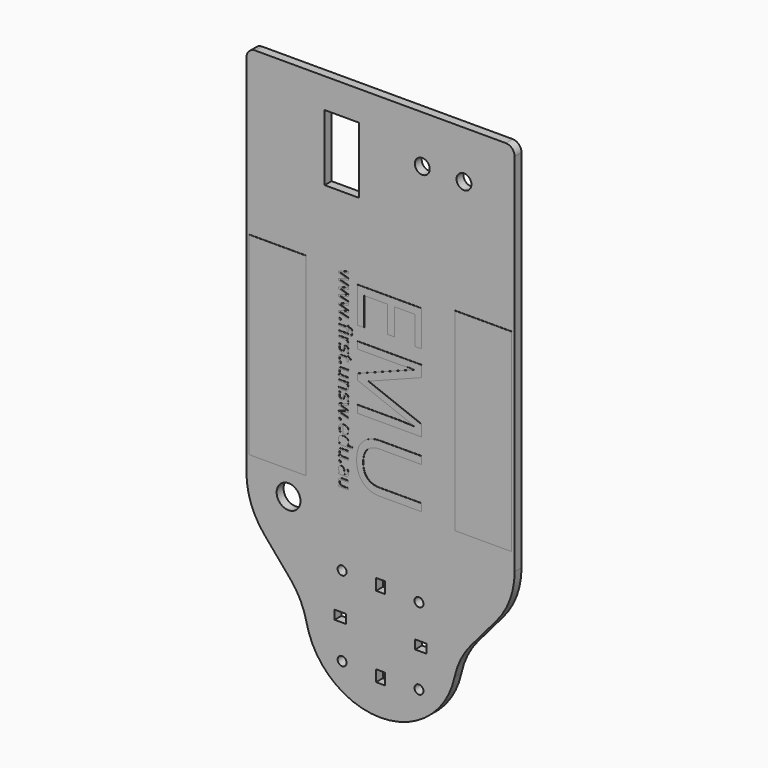
from build123d import *

# Parameters (mm, degrees)
F0_W      = 90
F0_H      = 135
F1_DEPTH  = 3
F2_R      = 2.5
F3_DEPTH  = 25.4
F4_R      = 25.4
F5_W      = 3.81
F5_H      = 1.5
F5_W_2    = 1.5
F5_H_2    = 3.81
F5_R      = 1.5
F6_DEPTH  = 25.4
F7_R      = 3
F9_DEPTH  = 25.4
F10_R     = 25.4
F12_DEPTH = 3
F13_R     = 1.5
F13_W     = 3.81
F13_H     = 3
F13_R_2   = 4
F13_W_2   = 3
F13_H_2   = 3.81
F13_W_3   = 3.2672184799
F13_H_3   = 0.4950909171
F13_W_4   = 11.5
F13_H_4   = 22.2
F13_R_3   = 2.5
F13_W_5   = 1
F13_H_5   = 65
F14_DEPTH = 0.1


# Not quite as in the source:
# - a feature names something its author has since deleted; it is built from what else it names


with BuildPart() as f1:
    # F0 (on Front) → F1 (new body)
    with BuildSketch(Plane.XZ):
        with Locations((-45, 67.5)):
            Rectangle(F0_W, F0_H)
        Polygon((-45, -70), (0, 0), (-90, 0), align=None)
    extrude(amount=F1_DEPTH)

    # F2 (on face) → F3 (cut)
    with BuildSketch(Plane.XZ.offset(3)):
        Polygon((-59, 125), (-63.75, 125), (-63.75, 119), (-58, 119), (-58, 125), align=None)
        Polygon((-58, 119), (-63.75, 119), (-63.75, 102.8), (-59, 102.8), (-58, 102.8), align=None)
        Polygon((-57, 125), (-58, 125), (-58, 119), (-52.25, 119), (-52.25, 125), align=None)
        Polygon((-52.25, 119), (-58, 119), (-58, 102.8), (-57, 102.8), (-52.25, 102.8), align=None)
        with Locations((-31, 119)):
            Circle(F2_R)
        with Locations((-17, 119)):
            Circle(F2_R)
    extrude(amount=-F3_DEPTH, mode=Mode.SUBTRACT)

    # F4
    f4_edges = [f1.edges().sort_by_distance(p)[0] for p in [
        (-45, -1.5, -70),
    ]]
    fillet(f4_edges, radius=F4_R)

    # F5 (on face) → F6 (cut)
    with BuildSketch(Plane.XZ.offset(3)):
        with Locations((-58.495, -22.2788609758)):
            Rectangle(F5_W, F5_H)
        with Locations((-58.495, -23.7788609758)):
            Rectangle(F5_W, F5_H)
        with Locations((-31.505, -22.2788609758)):
            Rectangle(F5_W, F5_H)
        with Locations((-31.505, -23.7788609758)):
            Rectangle(F5_W, F5_H)
        with Locations((-44.25, -36.5238609758)):
            Rectangle(F5_W_2, F5_H_2)
        with Locations((-45.75, -36.5238609758)):
            Rectangle(F5_W_2, F5_H_2)
        with Locations((-44.25, -9.5338609758)):
            Rectangle(F5_W_2, F5_H_2)
        with Locations((-45.75, -9.5338609758)):
            Rectangle(F5_W_2, F5_H_2)
        with Locations((-57.9, -9.1288609758)):
            Circle(F5_R)
        with Locations((-32.1, -10.1288609758)):
            Circle(F5_R)
        with Locations((-32.1, -35.9288609758)):
            Circle(F5_R)
        with Locations((-57.9, -35.9288609758)):
            Circle(F5_R)
    extrude(amount=-F6_DEPTH, mode=Mode.SUBTRACT)

    # F7
    f7_edges = [f1.edges().sort_by_distance(p)[0] for p in [
        (0, -1.5, 135),
        (-90, -1.5, 135),
    ]]
    fillet(f7_edges, radius=F7_R)

    # F8 (on face) → F9 (cut)
    with BuildSketch(Plane.XZ.offset(3)):
        with BuildLine():
            ThreePointArc((-66.3659332746, -36.7641037951), (-69.3706247886, -30.1865594475), (-70.4, -23.0288609758))
            Line((-70.4, -23.0288609758), (-90, 0))
            Line((-90, 0), (-66.3659332746, -36.7641037951))
        make_face()
        with BuildLine():
            Line((0, 0), (-19.6, -23.0288609758))
            ThreePointArc((-19.6, -23.0288609758), (-20.6293752114, -30.1865594475), (-23.6340667254, -36.7641037951))
            Line((-23.6340667254, -36.7641037951), (0, 0))
        make_face()
    extrude(amount=-F9_DEPTH, mode=Mode.SUBTRACT)

    # F10
    f10_edges = [f1.edges().sort_by_distance(p)[0] for p in [
        (-70.4, -1.5, -23.028861),
        (-90, -1.5, 0),
        (-19.6, -1.5, -23.028861),
        (0, -1.5, 0),
    ]]
    fillet(f10_edges, radius=F10_R)

    # F11 (on face) → F12 (cut)
    with BuildSketch(Plane.XZ.offset(3)):
        with BuildLine():
            ThreePointArc((-71.8725711956, 6.804616942), (-75.8725711956, 10.804616942), (-79.8725711956, 6.804616942))
            ThreePointArc((-79.8725711956, 6.804616942), (-75.8725711956, 2.804616942), (-71.8725711956, 6.804616942))
        make_face()
    extrude(amount=-F12_DEPTH, mode=Mode.SUBTRACT)

    # F13 (on face) → F14 (cut)
    with BuildSketch(Plane.XZ.offset(3)):
        with BuildLine():
            Line((-90, 132), (-90, 80))
            Line((-90, 80), (-89, 80))
            Line((-89, 80), (-70, 80))
            Line((-70, 80), (-70, 15))
            Line((-70, 15), (-89, 15))
            Line((-89, 15), (-90, 15))
            Line((-90, 15), (-90, 9.3457082747))
            ThreePointArc((-90, 9.3457082747), (-88.4376230462, 0.5748629616), (-83.9426986216, -7.1169771088))
            Line((-83.9426986216, -7.1169771088), (-75.3220457636, -17.2457432408))
            ThreePointArc((-75.3220457636, -17.2457432408), (-71.8878052771, -22.4669409617), (-69.8323721926, -28.3686448))
            ThreePointArc((-69.8323721926, -28.3686448), (-45, -48.4288609758), (-20.1676278074, -28.3686448))
            ThreePointArc((-20.1676278074, -28.3686448), (-18.1121947229, -22.4669409617), (-14.6779542364, -17.2457432408))
            Line((-14.6779542364, -17.2457432408), (-6.0573013784, -7.1169771088))
            ThreePointArc((-6.0573013784, -7.1169771088), (-1.5623769538, 0.5748629616), (0, 9.3457082747))
            Line((0, 9.3457082747), (0, 15))
            Line((0, 15), (-1, 15))
            Line((-1, 15), (-20, 15))
            Line((-20, 15), (-20, 80))
            Line((-20, 80), (-1, 80))
            Line((-1, 80), (0, 80))
            Line((0, 80), (0, 132))
            ThreePointArc((0, 132), (-0.8786796564, 134.1213203436), (-3, 135))
            Line((-3, 135), (-87, 135))
            ThreePointArc((-87, 135), (-89.1213203436, 134.1213203436), (-90, 132))
        make_face()
        with Locations((-57.9, -35.9288609758)):
            Circle(F13_R, mode=Mode.SUBTRACT)
        with Locations((-58.495, -23.0288609758)):
            Rectangle(F13_W, F13_H, mode=Mode.SUBTRACT)
        with Locations((-57.9, -9.1288609758)):
            Circle(F13_R, mode=Mode.SUBTRACT)
        with Locations((-75.8725711956, 6.804616942)):
            Circle(F13_R_2, mode=Mode.SUBTRACT)
        with BuildLine():
            Line((-55.7327815201, 18.1288982815), (-55.7327815201, 17.6280837699))
            Line((-55.7327815201, 17.6280837699), (-57.8524193193, 17.6280837699))
            add(Edge.make_bspline(
                [(-57.8524193193, 17.6280837699), (-58.2521169961, 17.6280837699), (-58.4486270711, 17.4463596472)],
                knots=[0, 0, 0, 1, 1, 1], degree=2))
            add(Edge.make_bspline(
                [(-58.4486270711, 17.4463596472), (-58.6451371461, 17.2646355244), (-58.6451371461, 16.8773389689)],
                knots=[0, 0, 0, 1, 1, 1], degree=2))
            add(Edge.make_bspline(
                [(-58.6451371461, 16.8773389689), (-58.6451371461, 16.3641233361), (-58.3651579859, 16.1275481002)],
                knots=[0, 0, 0, 1, 1, 1], degree=2))
            add(Edge.make_bspline(
                [(-58.3651579859, 16.1275481002), (-58.0851788256, 15.8909728643), (-57.4498598453, 15.8909728643)],
                knots=[0, 0, 0, 1, 1, 1], degree=2))
            Line((-57.4498598453, 15.8909728643), (-55.7327815201, 15.8909728643))
            Line((-55.7327815201, 15.8909728643), (-55.7327815201, 15.3958819472))
            Line((-55.7327815201, 15.3958819472), (-59, 15.3958819472))
            Line((-59, 15.3958819472), (-59, 15.8041650156))
            Line((-59, 15.8041650156), (-58.5621450271, 15.8757099458))
            Line((-58.5621450271, 15.8757099458), (-58.5621450271, 15.9024200531))
            add(Edge.make_bspline(
                [(-58.5621450271, 15.9024200531), (-58.803489925, 16.0540953052), (-58.9317938332, 16.3240581752)],
                knots=[0, 0, 0, 1, 1, 1], degree=2))
            add(Edge.make_bspline(
                [(-58.9317938332, 16.3240581752), (-59.0600977414, 16.5940210452), (-59.0600977414, 16.9402985075)],
                knots=[0, 0, 0, 1, 1, 1], degree=2))
            add(Edge.make_bspline(
                [(-59.0600977414, 16.9402985075), (-59.0600977414, 17.5365062593), (-58.7767798177, 17.8327022704)],
                knots=[0, 0, 0, 1, 1, 1], degree=2))
            add(Edge.make_bspline(
                [(-58.7767798177, 17.8327022704), (-58.4934618941, 18.1288982815), (-57.870544035, 18.1288982815)],
                knots=[0, 0, 0, 1, 1, 1], degree=2))
            Line((-57.870544035, 18.1288982815), (-55.7327815201, 18.1288982815))
        make_face(mode=Mode.SUBTRACT)
        with BuildLine():
            add(Edge.make_bspline(
                [(-58.992845507, 23.0850540806), (-58.8988831653, 23.1847400167), (-58.6842483746, 23.1847400167)],
                knots=[0, 0, 0, 1, 1, 1], degree=2))
            add(Edge.make_bspline(
                [(-58.6842483746, 23.1847400167), (-58.48392257, 23.1847400167), (-58.3813748367, 23.0936394723)],
                knots=[0, 0, 0, 1, 1, 1], degree=2))
            add(Edge.make_bspline(
                [(-58.3813748367, 23.0936394723), (-58.2788271034, 23.0025389278), (-58.2788271034, 22.8327389601)],
                knots=[0, 0, 0, 1, 1, 1], degree=2))
            add(Edge.make_bspline(
                [(-58.2788271034, 22.8327389601), (-58.2788271034, 22.6600771951), (-58.3813748367, 22.5632530563)],
                knots=[0, 0, 0, 1, 1, 1], degree=2))
            add(Edge.make_bspline(
                [(-58.3813748367, 22.5632530563), (-58.48392257, 22.4664289174), (-58.6842483746, 22.4664289174)],
                knots=[0, 0, 0, 1, 1, 1], degree=2))
            add(Edge.make_bspline(
                [(-58.6842483746, 22.4664289174), (-58.8778966524, 22.4664289174), (-58.9823522505, 22.5646839549)],
                knots=[0, 0, 0, 1, 1, 1], degree=2))
            add(Edge.make_bspline(
                [(-58.9823522505, 22.5646839549), (-59.0868078487, 22.6629389924), (-59.0868078487, 22.8327389601)],
                knots=[0, 0, 0, 1, 1, 1], degree=2))
            add(Edge.make_bspline(
                [(-59.0868078487, 22.8327389601), (-59.0868078487, 22.9853681445), (-58.992845507, 23.0850540806)],
                knots=[0, 0, 0, 1, 1, 1], degree=2))
        make_face(mode=Mode.SUBTRACT)
        with BuildLine():
            Line((-59, 19.1124025888), (-59, 19.4796665639))
            Line((-59, 19.4796665639), (-58.5344809874, 19.5779216014))
            Line((-58.5344809874, 19.5779216014), (-58.5344809874, 19.6017699115))
            add(Edge.make_bspline(
                [(-58.5344809874, 19.6017699115), (-58.8416472211, 19.8459766066), (-58.9508724813, 20.0887524032)],
                knots=[0, 0, 0, 1, 1, 1], degree=2))
            add(Edge.make_bspline(
                [(-58.9508724813, 20.0887524032), (-59.0600977414, 20.3315281997), (-59.0600977414, 20.6959303776)],
                knots=[0, 0, 0, 1, 1, 1], degree=2))
            add(Edge.make_bspline(
                [(-59.0600977414, 20.6959303776), (-59.0600977414, 21.1814819707), (-58.8092135194, 21.4571684351)],
                knots=[0, 0, 0, 1, 1, 1], degree=2))
            add(Edge.make_bspline(
                [(-58.8092135194, 21.4571684351), (-58.5583292975, 21.7328548995), (-58.0966260145, 21.7328548995)],
                knots=[0, 0, 0, 1, 1, 1], degree=2))
            add(Edge.make_bspline(
                [(-58.0966260145, 21.7328548995), (-57.1073981127, 21.7328548995), (-57.0597014925, 20.1502810432)],
                knots=[0, 0, 0, 1, 1, 1], degree=2))
            Line((-57.0597014925, 20.1502810432), (-57.0415767769, 19.5960463171))
            Line((-57.0415767769, 19.5960463171), (-56.8383891751, 19.5960463171))
            add(Edge.make_bspline(
                [(-56.8383891751, 19.5960463171), (-56.4539544167, 19.5960463171), (-56.2707993954, 19.7610766228)],
                knots=[0, 0, 0, 1, 1, 1], degree=2))
            add(Edge.make_bspline(
                [(-56.2707993954, 19.7610766228), (-56.087644374, 19.9261069285), (-56.087644374, 20.2905091064)],
                knots=[0, 0, 0, 1, 1, 1], degree=2))
            add(Edge.make_bspline(
                [(-56.087644374, 20.2905091064), (-56.087644374, 20.6987921748), (-56.3375746636, 21.2139156724)],
                knots=[0, 0, 0, 1, 1, 1], degree=2))
            Line((-56.3375746636, 21.2139156724), (-55.9588634996, 21.3665448568))
            add(Edge.make_bspline(
                [(-55.9588634996, 21.3665448568), (-55.8281747604, 21.1251999589), (-55.753768033, 20.8375893394)],
                knots=[0, 0, 0, 1, 1, 1], degree=2))
            add(Edge.make_bspline(
                [(-55.753768033, 20.8375893394), (-55.6793613056, 20.54997872), (-55.6793613056, 20.2599832695)],
                knots=[0, 0, 0, 1, 1, 1], degree=2))
            add(Edge.make_bspline(
                [(-55.6793613056, 20.2599832695), (-55.6793613056, 19.6761766389), (-55.9383539529, 19.3942896139)],
                knots=[0, 0, 0, 1, 1, 1], degree=2))
            add(Edge.make_bspline(
                [(-55.9383539529, 19.3942896139), (-56.1973466003, 19.1124025888), (-56.7697060421, 19.1124025888)],
                knots=[0, 0, 0, 1, 1, 1], degree=2))
            Line((-56.7697060421, 19.1124025888), (-59, 19.1124025888))
        make_face(mode=Mode.SUBTRACT)
        with BuildLine():
            Line((-55.7327815201, 26.8955370639), (-55.7327815201, 26.3947225524))
            Line((-55.7327815201, 26.3947225524), (-57.8524193193, 26.3947225524))
            add(Edge.make_bspline(
                [(-57.8524193193, 26.3947225524), (-58.2521169961, 26.3947225524), (-58.4486270711, 26.2129984297)],
                knots=[0, 0, 0, 1, 1, 1], degree=2))
            add(Edge.make_bspline(
                [(-58.4486270711, 26.2129984297), (-58.6451371461, 26.0312743069), (-58.6451371461, 25.6439777514)],
                knots=[0, 0, 0, 1, 1, 1], degree=2))
            add(Edge.make_bspline(
                [(-58.6451371461, 25.6439777514), (-58.6451371461, 25.1307621186), (-58.3651579859, 24.8941868827)],
                knots=[0, 0, 0, 1, 1, 1], degree=2))
            add(Edge.make_bspline(
                [(-58.3651579859, 24.8941868827), (-58.0851788256, 24.6576116468), (-57.4498598453, 24.6576116468)],
                knots=[0, 0, 0, 1, 1, 1], degree=2))
            Line((-57.4498598453, 24.6576116468), (-55.7327815201, 24.6576116468))
            Line((-55.7327815201, 24.6576116468), (-55.7327815201, 24.1625207297))
            Line((-55.7327815201, 24.1625207297), (-59, 24.1625207297))
            Line((-59, 24.1625207297), (-59, 24.5708037981))
            Line((-59, 24.5708037981), (-58.5621450271, 24.6423487283))
            Line((-58.5621450271, 24.6423487283), (-58.5621450271, 24.6690588356))
            add(Edge.make_bspline(
                [(-58.5621450271, 24.6690588356), (-58.803489925, 24.8207340877), (-58.9317938332, 25.0906969577)],
                knots=[0, 0, 0, 1, 1, 1], degree=2))
            add(Edge.make_bspline(
                [(-58.9317938332, 25.0906969577), (-59.0600977414, 25.3606598277), (-59.0600977414, 25.70693729)],
                knots=[0, 0, 0, 1, 1, 1], degree=2))
            add(Edge.make_bspline(
                [(-59.0600977414, 25.70693729), (-59.0600977414, 26.3031450418), (-58.7767798177, 26.5993410528)],
                knots=[0, 0, 0, 1, 1, 1], degree=2))
            add(Edge.make_bspline(
                [(-58.7767798177, 26.5993410528), (-58.4934618941, 26.8955370639), (-57.870544035, 26.8955370639)],
                knots=[0, 0, 0, 1, 1, 1], degree=2))
            Line((-57.870544035, 26.8955370639), (-55.7327815201, 26.8955370639))
        make_face(mode=Mode.SUBTRACT)
        with BuildLine():
            Line((-59, 28.3121266822), (-58.5621450271, 28.377948018))
            Line((-58.5621450271, 28.377948018), (-58.5621450271, 28.4046581253))
            add(Edge.make_bspline(
                [(-58.5621450271, 28.4046581253), (-59.0600977414, 28.7471198579), (-59.0600977414, 29.4301354584)],
                knots=[0, 0, 0, 1, 1, 1], degree=2))
            add(Edge.make_bspline(
                [(-59.0600977414, 29.4301354584), (-59.0600977414, 30.0711780331), (-58.6217658023, 30.4274717856)],
                knots=[0, 0, 0, 1, 1, 1], degree=2))
            add(Edge.make_bspline(
                [(-58.6217658023, 30.4274717856), (-58.1834338631, 30.7837655381), (-57.3754531179, 30.7837655381)],
                knots=[0, 0, 0, 1, 1, 1], degree=2))
            add(Edge.make_bspline(
                [(-57.3754531179, 30.7837655381), (-56.5674723727, 30.7837655381), (-56.1200780757, 30.426040887)],
                knots=[0, 0, 0, 1, 1, 1], degree=2))
            add(Edge.make_bspline(
                [(-56.1200780757, 30.426040887), (-55.6726837787, 30.0683162359), (-55.6726837787, 29.4301354584)],
                knots=[0, 0, 0, 1, 1, 1], degree=2))
            add(Edge.make_bspline(
                [(-55.6726837787, 29.4301354584), (-55.6726837787, 28.7652445736), (-56.156327507, 28.4103817197)],
                knots=[0, 0, 0, 1, 1, 1], degree=2))
            Line((-56.156327507, 28.4103817197), (-56.156327507, 28.3712704912))
            Line((-56.156327507, 28.3712704912), (-55.9207062035, 28.3922570041))
            Line((-55.9207062035, 28.3922570041), (-55.6908084944, 28.4046581253))
            Line((-55.6908084944, 28.4046581253), (-54.3610267248, 28.4046581253))
            Line((-54.3610267248, 28.4046581253), (-54.3610267248, 27.9095672082))
            Line((-54.3610267248, 27.9095672082), (-59, 27.9095672082))
            Line((-59, 27.9095672082), (-59, 28.3121266822))
        make_face(mode=Mode.SUBTRACT)
        with BuildLine():
            add(Edge.make_bspline(
                [(-59.0104932564, 32.0820675384), (-59.0600977414, 32.3157809771), (-59.0600977414, 32.6467955209)],
                knots=[0, 0, 0, 1, 1, 1], degree=2))
            add(Edge.make_bspline(
                [(-59.0600977414, 32.6467955209), (-59.0600977414, 33.3708302147), (-58.6184270388, 33.7900835058)],
                knots=[0, 0, 0, 1, 1, 1], degree=2))
            add(Edge.make_bspline(
                [(-58.6184270388, 33.7900835058), (-58.1767563363, 34.2093367968), (-57.3935778335, 34.2093367968)],
                knots=[0, 0, 0, 1, 1, 1], degree=2))
            add(Edge.make_bspline(
                [(-57.3935778335, 34.2093367968), (-56.6027678716, 34.2093367968), (-56.1377258252, 33.8201323765)],
                knots=[0, 0, 0, 1, 1, 1], degree=2))
            add(Edge.make_bspline(
                [(-56.1377258252, 33.8201323765), (-55.6726837787, 33.4309279561), (-55.6726837787, 32.7746224629)],
                knots=[0, 0, 0, 1, 1, 1], degree=2))
            add(Edge.make_bspline(
                [(-55.6726837787, 32.7746224629), (-55.6726837787, 32.1612439279), (-56.0766741514, 31.8035192768)],
                knots=[0, 0, 0, 1, 1, 1], degree=2))
            add(Edge.make_bspline(
                [(-56.0766741514, 31.8035192768), (-56.480664524, 31.4457946257), (-57.1426936116, 31.4457946257)],
                knots=[0, 0, 0, 1, 1, 1], degree=2))
            Line((-57.1426936116, 31.4457946257), (-57.4555834397, 31.4457946257))
            Line((-57.4555834397, 31.4457946257), (-57.4555834397, 33.6961211641))
            add(Edge.make_bspline(
                [(-57.4555834397, 33.6961211641), (-58.0308046787, 33.6808582456), (-58.3289085546, 33.4051717812)],
                knots=[0, 0, 0, 1, 1, 1], degree=2))
            add(Edge.make_bspline(
                [(-58.3289085546, 33.4051717812), (-58.6270124305, 33.1294853168), (-58.6270124305, 32.6286708053)],
                knots=[0, 0, 0, 1, 1, 1], degree=2))
            add(Edge.make_bspline(
                [(-58.6270124305, 32.6286708053), (-58.6270124305, 32.1011461865), (-58.4066540454, 31.5860226889)],
                knots=[0, 0, 0, 1, 1, 1], degree=2))
            Line((-58.4066540454, 31.5860226889), (-58.8483247479, 31.5860226889))
            add(Edge.make_bspline(
                [(-58.8483247479, 31.5860226889), (-58.9608887715, 31.8483540997), (-59.0104932564, 32.0820675384)],
                knots=[0, 0, 0, 1, 1, 1], degree=2))
        make_face(mode=Mode.SUBTRACT)
        with BuildLine():
            add(Edge.make_bspline(
                [(-58.992845507, 35.6235415841), (-58.8988831653, 35.7232275202), (-58.6842483746, 35.7232275202)],
                knots=[0, 0, 0, 1, 1, 1], degree=2))
            add(Edge.make_bspline(
                [(-58.6842483746, 35.7232275202), (-58.48392257, 35.7232275202), (-58.3813748367, 35.6321269757)],
                knots=[0, 0, 0, 1, 1, 1], degree=2))
            add(Edge.make_bspline(
                [(-58.3813748367, 35.6321269757), (-58.2788271034, 35.5410264313), (-58.2788271034, 35.3712264636)],
                knots=[0, 0, 0, 1, 1, 1], degree=2))
            add(Edge.make_bspline(
                [(-58.2788271034, 35.3712264636), (-58.2788271034, 35.1985646986), (-58.3813748367, 35.1017405597)],
                knots=[0, 0, 0, 1, 1, 1], degree=2))
            add(Edge.make_bspline(
                [(-58.3813748367, 35.1017405597), (-58.48392257, 35.0049164208), (-58.6842483746, 35.0049164208)],
                knots=[0, 0, 0, 1, 1, 1], degree=2))
            add(Edge.make_bspline(
                [(-58.6842483746, 35.0049164208), (-58.8778966524, 35.0049164208), (-58.9823522505, 35.1031714583)],
                knots=[0, 0, 0, 1, 1, 1], degree=2))
            add(Edge.make_bspline(
                [(-58.9823522505, 35.1031714583), (-59.0868078487, 35.2014264958), (-59.0868078487, 35.3712264636)],
                knots=[0, 0, 0, 1, 1, 1], degree=2))
            add(Edge.make_bspline(
                [(-59.0868078487, 35.3712264636), (-59.0868078487, 35.523855648), (-58.992845507, 35.6235415841)],
                knots=[0, 0, 0, 1, 1, 1], degree=2))
        make_face(mode=Mode.SUBTRACT)
        with BuildLine():
            Line((-59, 37.1445868005), (-59, 37.7322091607))
            Line((-59, 37.7322091607), (-57.0835498026, 38.3312787097))
            add(Edge.make_bspline(
                [(-57.0835498026, 38.3312787097), (-56.9070723081, 38.3885146539), (-56.284154449, 38.5430517031)],
                knots=[0, 0, 0, 1, 1, 1], degree=2))
            Line((-56.284154449, 38.5430517031), (-56.284154449, 38.5669000132))
            add(Edge.make_bspline(
                [(-56.284154449, 38.5669000132), (-56.8059554734, 38.6861415636), (-57.089273397, 38.7758112094)],
                knots=[0, 0, 0, 1, 1, 1], degree=2))
            Line((-57.089273397, 38.7758112094), (-59, 39.3930054741))
            Line((-59, 39.3930054741), (-59, 39.9653649158))
            Line((-59, 39.9653649158), (-55.7327815201, 40.8563377801))
            Line((-55.7327815201, 40.8563377801), (-55.7327815201, 40.337398553))
            add(Edge.make_bspline(
                [(-55.7327815201, 40.337398553), (-56.9643082522, 40.0216469276), (-57.6082126242, 39.8561396557)],
                knots=[0, 0, 0, 1, 1, 1], degree=2))
            add(Edge.make_bspline(
                [(-57.6082126242, 39.8561396557), (-58.2521169961, 39.6906323838), (-58.4753371784, 39.6667840737)],
                knots=[0, 0, 0, 1, 1, 1], degree=2))
            Line((-58.4753371784, 39.6667840737), (-58.4753371784, 39.6429357637))
            add(Edge.make_bspline(
                [(-58.4753371784, 39.6429357637), (-58.3055372107, 39.610502062), (-58.0355743407, 39.5375262331)],
                knots=[0, 0, 0, 1, 1, 1], degree=2))
            add(Edge.make_bspline(
                [(-58.0355743407, 39.5375262331), (-57.7656114707, 39.4645504043), (-57.6082126242, 39.4101762574)],
                knots=[0, 0, 0, 1, 1, 1], degree=2))
            Line((-57.6082126242, 39.4101762574), (-55.7327815201, 38.8111067083))
            Line((-55.7327815201, 38.8111067083), (-55.7327815201, 38.2749966979))
            Line((-55.7327815201, 38.2749966979), (-57.6082126242, 37.690236135))
            add(Edge.make_bspline(
                [(-57.6082126242, 37.690236135), (-58.1204743245, 37.5232979645), (-58.469613584, 37.4641541555)],
                knots=[0, 0, 0, 1, 1, 1], degree=2))
            Line((-58.469613584, 37.4641541555), (-58.469613584, 37.4403058454))
            add(Edge.make_bspline(
                [(-58.469613584, 37.4403058454), (-58.3618192225, 37.4279047242), (-58.138122074, 37.3759154082)],
                knots=[0, 0, 0, 1, 1, 1], degree=2))
            add(Edge.make_bspline(
                [(-58.138122074, 37.3759154082), (-57.9144249255, 37.3239260923), (-55.7327815201, 36.7544284477)],
                knots=[0, 0, 0, 1, 1, 1], degree=2))
            Line((-55.7327815201, 36.7544284477), (-55.7327815201, 36.2421667474))
            Line((-55.7327815201, 36.2421667474), (-59, 37.1445868005))
        make_face(mode=Mode.SUBTRACT)
        with BuildLine():
            add(Edge.make_bspline(
                [(-57.5691013957, 41.4096185738), (-57.7837361863, 41.2054770396), (-58.1090271357, 41.2054770396)],
                knots=[0, 0, 0, 1, 1, 1], degree=2))
            add(Edge.make_bspline(
                [(-58.1090271357, 41.2054770396), (-58.5650068243, 41.2054770396), (-58.8125522828, 41.545076975)],
                knots=[0, 0, 0, 1, 1, 1], degree=2))
            add(Edge.make_bspline(
                [(-58.8125522828, 41.545076975), (-59.0600977414, 41.8846769104), (-59.0600977414, 42.4990093779)],
                knots=[0, 0, 0, 1, 1, 1], degree=2))
            add(Edge.make_bspline(
                [(-59.0600977414, 42.4990093779), (-59.0600977414, 43.1486373443), (-58.8540483424, 43.5120855898)],
                knots=[0, 0, 0, 1, 1, 1], degree=2))
            Line((-58.8540483424, 43.5120855898), (-58.3952068566, 43.5120855898))
            add(Edge.make_bspline(
                [(-58.3952068566, 43.5120855898), (-58.5144484069, 43.2764642862), (-58.5826545737, 43.0069783824)],
                knots=[0, 0, 0, 1, 1, 1], degree=2))
            add(Edge.make_bspline(
                [(-58.5826545737, 43.0069783824), (-58.6508607405, 42.7374924786), (-58.6508607405, 42.4866082567)],
                knots=[0, 0, 0, 1, 1, 1], degree=2))
            add(Edge.make_bspline(
                [(-58.6508607405, 42.4866082567), (-58.6508607405, 42.0993117011), (-58.5273264944, 41.8908774711)],
                knots=[0, 0, 0, 1, 1, 1], degree=2))
            add(Edge.make_bspline(
                [(-58.5273264944, 41.8908774711), (-58.4037922482, 41.682443241), (-58.150046229, 41.682443241)],
                knots=[0, 0, 0, 1, 1, 1], degree=2))
            add(Edge.make_bspline(
                [(-58.150046229, 41.682443241), (-57.9592597485, 41.682443241), (-57.8238013472, 41.8474735467)],
                knots=[0, 0, 0, 1, 1, 1], degree=2))
            add(Edge.make_bspline(
                [(-57.8238013472, 41.8474735467), (-57.688342946, 42.0125038524), (-57.5032800599, 42.4932857835)],
                knots=[0, 0, 0, 1, 1, 1], degree=2))
            add(Edge.make_bspline(
                [(-57.5032800599, 42.4932857835), (-57.3334800922, 42.949265472), (-57.2066070826, 43.1414828512)],
                knots=[0, 0, 0, 1, 1, 1], degree=2))
            add(Edge.make_bspline(
                [(-57.2066070826, 43.1414828512), (-57.079734073, 43.3337002304), (-56.9189964631, 43.4276625721)],
                knots=[0, 0, 0, 1, 1, 1], degree=2))
            add(Edge.make_bspline(
                [(-56.9189964631, 43.4276625721), (-56.7582588532, 43.5216249138), (-56.535038671, 43.5216249138)],
                knots=[0, 0, 0, 1, 1, 1], degree=2))
            add(Edge.make_bspline(
                [(-56.535038671, 43.5216249138), (-56.1353409941, 43.5216249138), (-55.9040123864, 43.1963339644)],
                knots=[0, 0, 0, 1, 1, 1], degree=2))
            add(Edge.make_bspline(
                [(-55.9040123864, 43.1963339644), (-55.6726837787, 42.871043015), (-55.6726837787, 42.3053611001)],
                knots=[0, 0, 0, 1, 1, 1], degree=2))
            add(Edge.make_bspline(
                [(-55.6726837787, 42.3053611001), (-55.6726837787, 41.7778364813), (-55.8873185694, 41.2732062402)],
                knots=[0, 0, 0, 1, 1, 1], degree=2))
            Line((-55.8873185694, 41.2732062402), (-56.2898780434, 41.4496837347))
            add(Edge.make_bspline(
                [(-56.2898780434, 41.4496837347), (-56.087644374, 41.9409589222), (-56.087644374, 42.340656599)],
                knots=[0, 0, 0, 1, 1, 1], degree=2))
            add(Edge.make_bspline(
                [(-56.087644374, 42.340656599), (-56.087644374, 42.6926576557), (-56.1978235665, 42.8715199812)],
                knots=[0, 0, 0, 1, 1, 1], degree=2))
            add(Edge.make_bspline(
                [(-56.1978235665, 42.8715199812), (-56.3080027591, 43.0503823068), (-56.5016510369, 43.0503823068)],
                knots=[0, 0, 0, 1, 1, 1], degree=2))
            add(Edge.make_bspline(
                [(-56.5016510369, 43.0503823068), (-56.6332937084, 43.0503823068), (-56.7253481853, 42.9831300724)],
                knots=[0, 0, 0, 1, 1, 1], degree=2))
            add(Edge.make_bspline(
                [(-56.7253481853, 42.9831300724), (-56.8174026622, 42.9158778379), (-56.9008717475, 42.7670643831)],
                knots=[0, 0, 0, 1, 1, 1], degree=2))
            add(Edge.make_bspline(
                [(-56.9008717475, 42.7670643831), (-56.9843408327, 42.6182509282), (-57.1426936116, 42.1947049414)],
                knots=[0, 0, 0, 1, 1, 1], degree=2))
            add(Edge.make_bspline(
                [(-57.1426936116, 42.1947049414), (-57.354466605, 41.613760108), (-57.5691013957, 41.4096185738)],
                knots=[0, 0, 0, 1, 1, 1], degree=2))
        make_face(mode=Mode.SUBTRACT)
        with Locations((-45, -36.5238609758)):
            Rectangle(F13_W_2, F13_H_2, mode=Mode.SUBTRACT)
        with Locations((-32.1, -35.9288609758)):
            Circle(F13_R, mode=Mode.SUBTRACT)
        with Locations((-45, -9.5338609758)):
            Rectangle(F13_W_2, F13_H_2, mode=Mode.SUBTRACT)
        with Locations((-31.505, -23.0288609758)):
            Rectangle(F13_W, F13_H, mode=Mode.SUBTRACT)
        with Locations((-32.1, -10.1288609758)):
            Circle(F13_R, mode=Mode.SUBTRACT)
        with BuildLine():
            Line((-31.18329718, 19.446131598), (-31.18329718, 16.9504699928))
            Line((-31.18329718, 16.9504699928), (-45.0762834418, 16.9504699928))
            add(Edge.make_bspline(
                [(-45.0762834418, 16.9504699928), (-48.751626898, 16.9504699928), (-50.852494577, 19.1688358641)],
                knots=[0, 0, 0, 1, 1, 1], degree=2))
            add(Edge.make_bspline(
                [(-50.852494577, 19.1688358641), (-52.953362256, 21.3872017354), (-52.953362256, 25.2646420824)],
                knots=[0, 0, 0, 1, 1, 1], degree=2))
            add(Edge.make_bspline(
                [(-52.953362256, 25.2646420824), (-52.953362256, 29.1420824295), (-50.8360448301, 31.2640997831)],
                knots=[0, 0, 0, 1, 1, 1], degree=2))
            add(Edge.make_bspline(
                [(-50.8360448301, 31.2640997831), (-48.7187274042, 33.3861171367), (-45.0198843095, 33.3861171367)],
                knots=[0, 0, 0, 1, 1, 1], degree=2))
            Line((-45.0198843095, 33.3861171367), (-31.18329718, 33.3861171367))
            Line((-31.18329718, 33.3861171367), (-31.18329718, 30.8857556038))
            Line((-31.18329718, 30.8857556038), (-45.1937816341, 30.8857556038))
            add(Edge.make_bspline(
                [(-45.1937816341, 30.8857556038), (-47.8821402748, 30.8857556038), (-49.3226681128, 29.4170281996)],
                knots=[0, 0, 0, 1, 1, 1], degree=2))
            add(Edge.make_bspline(
                [(-49.3226681128, 29.4170281996), (-50.7631959508, 27.9483007954), (-50.7631959508, 25.1001446132)],
                knots=[0, 0, 0, 1, 1, 1], degree=2))
            add(Edge.make_bspline(
                [(-50.7631959508, 25.1001446132), (-50.7631959508, 22.3835864064), (-49.3156182213, 20.9148590022)],
                knots=[0, 0, 0, 1, 1, 1], degree=2))
            add(Edge.make_bspline(
                [(-49.3156182213, 20.9148590022), (-47.8680404917, 19.446131598), (-45.165582068, 19.446131598)],
                knots=[0, 0, 0, 1, 1, 1], degree=2))
            Line((-45.165582068, 19.446131598), (-31.18329718, 19.446131598))
        make_face(mode=Mode.SUBTRACT)
        with BuildLine():
            Line((-59, 44.3286517266), (-59, 44.8237426437))
            Line((-59, 44.8237426437), (-56.8860857952, 44.8237426437))
            add(Edge.make_bspline(
                [(-56.8860857952, 44.8237426437), (-56.4873420508, 44.8237426437), (-56.2903550096, 45.0054667665)],
                knots=[0, 0, 0, 1, 1, 1], degree=2))
            add(Edge.make_bspline(
                [(-56.2903550096, 45.0054667665), (-56.0933679684, 45.1871908892), (-56.0933679684, 45.5754413772)],
                knots=[0, 0, 0, 1, 1, 1], degree=2))
            add(Edge.make_bspline(
                [(-56.0933679684, 45.5754413772), (-56.0933679684, 46.0877030775), (-56.3704853315, 46.3261861783)],
                knots=[0, 0, 0, 1, 1, 1], degree=2))
            add(Edge.make_bspline(
                [(-56.3704853315, 46.3261861783), (-56.6476026945, 46.564669279), (-57.285783472, 46.564669279)],
                knots=[0, 0, 0, 1, 1, 1], degree=2))
            Line((-57.285783472, 46.564669279), (-59, 46.564669279))
            Line((-59, 46.564669279), (-59, 47.0597601961))
            Line((-59, 47.0597601961), (-55.7327815201, 47.0597601961))
            Line((-55.7327815201, 47.0597601961), (-55.7327815201, 46.6572007221))
            Line((-55.7327815201, 46.6572007221), (-56.1801758171, 46.5770704002))
            Line((-56.1801758171, 46.5770704002), (-56.1801758171, 46.5532220901))
            add(Edge.make_bspline(
                [(-56.1801758171, 46.5532220901), (-55.9388309192, 46.4005929057), (-55.8057573489, 46.1263373398)],
                knots=[0, 0, 0, 1, 1, 1], degree=2))
            add(Edge.make_bspline(
                [(-55.8057573489, 46.1263373398), (-55.6726837787, 45.852081774), (-55.6726837787, 45.5153436358)],
                knots=[0, 0, 0, 1, 1, 1], degree=2))
            add(Edge.make_bspline(
                [(-55.6726837787, 45.5153436358), (-55.6726837787, 44.9248594784), (-55.957432601, 44.6267556025)],
                knots=[0, 0, 0, 1, 1, 1], degree=2))
            add(Edge.make_bspline(
                [(-55.957432601, 44.6267556025), (-56.2421814233, 44.3286517266), (-56.868915012, 44.3286517266)],
                knots=[0, 0, 0, 1, 1, 1], degree=2))
            Line((-56.868915012, 44.3286517266), (-59, 44.3286517266))
        make_face(mode=Mode.SUBTRACT)
        with BuildLine():
            Line((-55.7327815201, 50.8421021735), (-55.7327815201, 50.341287662))
            Line((-55.7327815201, 50.341287662), (-57.8524193193, 50.341287662))
            add(Edge.make_bspline(
                [(-57.8524193193, 50.341287662), (-58.2521169961, 50.341287662), (-58.4486270711, 50.1595635392)],
                knots=[0, 0, 0, 1, 1, 1], degree=2))
            add(Edge.make_bspline(
                [(-58.4486270711, 50.1595635392), (-58.6451371461, 49.9778394165), (-58.6451371461, 49.5905428609)],
                knots=[0, 0, 0, 1, 1, 1], degree=2))
            add(Edge.make_bspline(
                [(-58.6451371461, 49.5905428609), (-58.6451371461, 49.0773272282), (-58.3651579859, 48.8407519923)],
                knots=[0, 0, 0, 1, 1, 1], degree=2))
            add(Edge.make_bspline(
                [(-58.3651579859, 48.8407519923), (-58.0851788256, 48.6041767563), (-57.4498598453, 48.6041767563)],
                knots=[0, 0, 0, 1, 1, 1], degree=2))
            Line((-57.4498598453, 48.6041767563), (-55.7327815201, 48.6041767563))
            Line((-55.7327815201, 48.6041767563), (-55.7327815201, 48.1090858392))
            Line((-55.7327815201, 48.1090858392), (-56.8021397438, 48.1090858392))
            Line((-56.8021397438, 48.1090858392), (-59, 48.1090858392))
            Line((-59, 48.1090858392), (-59, 48.5173689077))
            Line((-59, 48.5173689077), (-58.5621450271, 48.5889138379))
            Line((-58.5621450271, 48.5889138379), (-58.5621450271, 48.6156239452))
            add(Edge.make_bspline(
                [(-58.5621450271, 48.6156239452), (-58.803489925, 48.7672991972), (-58.9317938332, 49.0372620672)],
                knots=[0, 0, 0, 1, 1, 1], degree=2))
            add(Edge.make_bspline(
                [(-58.9317938332, 49.0372620672), (-59.0600977414, 49.3072249373), (-59.0600977414, 49.6535023995)],
                knots=[0, 0, 0, 1, 1, 1], degree=2))
            add(Edge.make_bspline(
                [(-59.0600977414, 49.6535023995), (-59.0600977414, 50.2497101513), (-58.7767798177, 50.5459061624)],
                knots=[0, 0, 0, 1, 1, 1], degree=2))
            add(Edge.make_bspline(
                [(-58.7767798177, 50.5459061624), (-58.4934618941, 50.8421021735), (-57.870544035, 50.8421021735)],
                knots=[0, 0, 0, 1, 1, 1], degree=2))
            Line((-57.870544035, 50.8421021735), (-55.7327815201, 50.8421021735))
        make_face(mode=Mode.SUBTRACT)
        with BuildLine():
            add(Edge.make_bspline(
                [(-58.992845507, 52.4032125508), (-58.8988831653, 52.5028984869), (-58.6842483746, 52.5028984869)],
                knots=[0, 0, 0, 1, 1, 1], degree=2))
            add(Edge.make_bspline(
                [(-58.6842483746, 52.5028984869), (-58.48392257, 52.5028984869), (-58.3813748367, 52.4117979424)],
                knots=[0, 0, 0, 1, 1, 1], degree=2))
            add(Edge.make_bspline(
                [(-58.3813748367, 52.4117979424), (-58.2788271034, 52.320697398), (-58.2788271034, 52.1508974303)],
                knots=[0, 0, 0, 1, 1, 1], degree=2))
            add(Edge.make_bspline(
                [(-58.2788271034, 52.1508974303), (-58.2788271034, 51.9782356653), (-58.3813748367, 51.8814115264)],
                knots=[0, 0, 0, 1, 1, 1], degree=2))
            add(Edge.make_bspline(
                [(-58.3813748367, 51.8814115264), (-58.48392257, 51.7845873875), (-58.6842483746, 51.7845873875)],
                knots=[0, 0, 0, 1, 1, 1], degree=2))
            add(Edge.make_bspline(
                [(-58.6842483746, 51.7845873875), (-58.8778966524, 51.7845873875), (-58.9823522505, 51.882842425)],
                knots=[0, 0, 0, 1, 1, 1], degree=2))
            add(Edge.make_bspline(
                [(-58.9823522505, 51.882842425), (-59.0868078487, 51.9810974625), (-59.0868078487, 52.1508974303)],
                knots=[0, 0, 0, 1, 1, 1], degree=2))
            add(Edge.make_bspline(
                [(-59.0868078487, 52.1508974303), (-59.0868078487, 52.3035266147), (-58.992845507, 52.4032125508)],
                knots=[0, 0, 0, 1, 1, 1], degree=2))
        make_face(mode=Mode.SUBTRACT)
        with BuildLine():
            add(Edge.make_bspline(
                [(-58.4929849279, 53.9156723756), (-58.6508607405, 53.7754443124), (-58.6508607405, 53.5312376172)],
                knots=[0, 0, 0, 1, 1, 1], degree=2))
            add(Edge.make_bspline(
                [(-58.6508607405, 53.5312376172), (-58.6508607405, 53.3995949456), (-58.6317820925, 53.2774915981)],
                knots=[0, 0, 0, 1, 1, 1], degree=2))
            add(Edge.make_bspline(
                [(-58.6317820925, 53.2774915981), (-58.6127034444, 53.1553882505), (-58.5917169316, 53.0838433203)],
                knots=[0, 0, 0, 1, 1, 1], degree=2))
            Line((-58.5917169316, 53.0838433203), (-58.9704280955, 53.0838433203))
            add(Edge.make_bspline(
                [(-58.9704280955, 53.0838433203), (-59.0085853916, 53.1639736421), (-59.0343415665, 53.3204185562)],
                knots=[0, 0, 0, 1, 1, 1], degree=2))
            add(Edge.make_bspline(
                [(-59.0343415665, 53.3204185562), (-59.0600977414, 53.4768634703), (-59.0600977414, 53.6027825474)],
                knots=[0, 0, 0, 1, 1, 1], degree=2))
            add(Edge.make_bspline(
                [(-59.0600977414, 53.6027825474), (-59.0600977414, 54.5500374235), (-58.0613305156, 54.5500374235)],
                knots=[0, 0, 0, 1, 1, 1], degree=2))
            Line((-58.0613305156, 54.5500374235), (-56.1172162785, 54.5500374235))
            Line((-56.1172162785, 54.5500374235), (-56.1172162785, 55.0184182333))
            Line((-56.1172162785, 55.0184182333), (-55.8787331778, 55.0184182333))
            Line((-55.8787331778, 55.0184182333), (-55.6726837787, 54.5500374235))
            Line((-55.6726837787, 54.5500374235), (-54.9753591922, 54.3420801597))
            Line((-54.9753591922, 54.3420801597), (-54.9753591922, 54.0559004388))
            Line((-54.9753591922, 54.0559004388), (-55.7327815201, 54.0559004388))
            Line((-55.7327815201, 54.0559004388), (-55.7327815201, 53.1076916303))
            Line((-55.7327815201, 53.1076916303), (-56.1172162785, 53.1076916303))
            Line((-56.1172162785, 53.1076916303), (-56.1172162785, 54.0559004388))
            Line((-56.1172162785, 54.0559004388), (-58.0403440027, 54.0559004388))
            add(Edge.make_bspline(
                [(-58.0403440027, 54.0559004388), (-58.3351091152, 54.0559004388), (-58.4929849279, 53.9156723756)],
                knots=[0, 0, 0, 1, 1, 1], degree=2))
        make_face(mode=Mode.SUBTRACT)
        with BuildLine():
            add(Edge.make_bspline(
                [(-57.5691013957, 55.5955473371), (-57.7837361863, 55.3914058028), (-58.1090271357, 55.3914058028)],
                knots=[0, 0, 0, 1, 1, 1], degree=2))
            add(Edge.make_bspline(
                [(-58.1090271357, 55.3914058028), (-58.5650068243, 55.3914058028), (-58.8125522828, 55.7310057383)],
                knots=[0, 0, 0, 1, 1, 1], degree=2))
            add(Edge.make_bspline(
                [(-58.8125522828, 55.7310057383), (-59.0600977414, 56.0706056737), (-59.0600977414, 56.6849381412)],
                knots=[0, 0, 0, 1, 1, 1], degree=2))
            add(Edge.make_bspline(
                [(-59.0600977414, 56.6849381412), (-59.0600977414, 57.3345661075), (-58.8540483424, 57.698014353)],
                knots=[0, 0, 0, 1, 1, 1], degree=2))
            Line((-58.8540483424, 57.698014353), (-58.3952068566, 57.698014353))
            add(Edge.make_bspline(
                [(-58.3952068566, 57.698014353), (-58.5144484069, 57.4623930495), (-58.5826545737, 57.1929071457)],
                knots=[0, 0, 0, 1, 1, 1], degree=2))
            add(Edge.make_bspline(
                [(-58.5826545737, 57.1929071457), (-58.6508607405, 56.9234212419), (-58.6508607405, 56.6725370199)],
                knots=[0, 0, 0, 1, 1, 1], degree=2))
            add(Edge.make_bspline(
                [(-58.6508607405, 56.6725370199), (-58.6508607405, 56.2852404643), (-58.5273264944, 56.0768062343)],
                knots=[0, 0, 0, 1, 1, 1], degree=2))
            add(Edge.make_bspline(
                [(-58.5273264944, 56.0768062343), (-58.4037922482, 55.8683720043), (-58.150046229, 55.8683720043)],
                knots=[0, 0, 0, 1, 1, 1], degree=2))
            add(Edge.make_bspline(
                [(-58.150046229, 55.8683720043), (-57.9592597485, 55.8683720043), (-57.8238013472, 56.03340231)],
                knots=[0, 0, 0, 1, 1, 1], degree=2))
            add(Edge.make_bspline(
                [(-57.8238013472, 56.03340231), (-57.688342946, 56.1984326157), (-57.5032800599, 56.6792145467)],
                knots=[0, 0, 0, 1, 1, 1], degree=2))
            add(Edge.make_bspline(
                [(-57.5032800599, 56.6792145467), (-57.3334800922, 57.1351942353), (-57.2066070826, 57.3274116145)],
                knots=[0, 0, 0, 1, 1, 1], degree=2))
            add(Edge.make_bspline(
                [(-57.2066070826, 57.3274116145), (-57.079734073, 57.5196289937), (-56.9189964631, 57.6135913354)],
                knots=[0, 0, 0, 1, 1, 1], degree=2))
            add(Edge.make_bspline(
                [(-56.9189964631, 57.6135913354), (-56.7582588532, 57.707553677), (-56.535038671, 57.707553677)],
                knots=[0, 0, 0, 1, 1, 1], degree=2))
            add(Edge.make_bspline(
                [(-56.535038671, 57.707553677), (-56.1353409941, 57.707553677), (-55.9040123864, 57.3822627277)],
                knots=[0, 0, 0, 1, 1, 1], degree=2))
            add(Edge.make_bspline(
                [(-55.9040123864, 57.3822627277), (-55.6726837787, 57.0569717783), (-55.6726837787, 56.4912898634)],
                knots=[0, 0, 0, 1, 1, 1], degree=2))
            add(Edge.make_bspline(
                [(-55.6726837787, 56.4912898634), (-55.6726837787, 55.9637652446), (-55.8873185694, 55.4591350034)],
                knots=[0, 0, 0, 1, 1, 1], degree=2))
            Line((-55.8873185694, 55.4591350034), (-56.2898780434, 55.635612498))
            add(Edge.make_bspline(
                [(-56.2898780434, 55.635612498), (-56.087644374, 56.1268876855), (-56.087644374, 56.5265853623)],
                knots=[0, 0, 0, 1, 1, 1], degree=2))
            add(Edge.make_bspline(
                [(-56.087644374, 56.5265853623), (-56.087644374, 56.8785864189), (-56.1978235665, 57.0574487445)],
                knots=[0, 0, 0, 1, 1, 1], degree=2))
            add(Edge.make_bspline(
                [(-56.1978235665, 57.0574487445), (-56.3080027591, 57.23631107), (-56.5016510369, 57.23631107)],
                knots=[0, 0, 0, 1, 1, 1], degree=2))
            add(Edge.make_bspline(
                [(-56.5016510369, 57.23631107), (-56.6332937084, 57.23631107), (-56.7253481853, 57.1690588356)],
                knots=[0, 0, 0, 1, 1, 1], degree=2))
            add(Edge.make_bspline(
                [(-56.7253481853, 57.1690588356), (-56.8174026622, 57.1018066012), (-56.9008717475, 56.9529931464)],
                knots=[0, 0, 0, 1, 1, 1], degree=2))
            add(Edge.make_bspline(
                [(-56.9008717475, 56.9529931464), (-56.9843408327, 56.8041796915), (-57.1426936116, 56.3806337046)],
                knots=[0, 0, 0, 1, 1, 1], degree=2))
            add(Edge.make_bspline(
                [(-57.1426936116, 56.3806337046), (-57.354466605, 55.7996888713), (-57.5691013957, 55.5955473371)],
                knots=[0, 0, 0, 1, 1, 1], degree=2))
        make_face(mode=Mode.SUBTRACT)
        with BuildLine():
            add(Edge.make_bspline(
                [(-55.8458225099, 59.0640455539), (-55.6726837787, 58.8074377376), (-55.6726837787, 58.5002715038)],
                knots=[0, 0, 0, 1, 1, 1], degree=2))
            add(Edge.make_bspline(
                [(-55.6726837787, 58.5002715038), (-55.6726837787, 58.282774916), (-55.7089332101, 58.1101131511)],
                knots=[0, 0, 0, 1, 1, 1], degree=2))
            Line((-55.7089332101, 58.1101131511), (-56.1677746958, 58.1787962841))
            add(Edge.make_bspline(
                [(-56.1677746958, 58.1787962841), (-56.1229398729, 58.3810299535), (-56.1229398729, 58.5365209351)],
                knots=[0, 0, 0, 1, 1, 1], degree=2))
            add(Edge.make_bspline(
                [(-56.1229398729, 58.5365209351), (-56.1229398729, 58.9333568147), (-56.4448920589, 59.2147668736)],
                knots=[0, 0, 0, 1, 1, 1], degree=2))
            add(Edge.make_bspline(
                [(-56.4448920589, 59.2147668736), (-56.7668442449, 59.4961769324), (-57.2466722435, 59.4961769324)],
                knots=[0, 0, 0, 1, 1, 1], degree=2))
            Line((-57.2466722435, 59.4961769324), (-59, 59.4961769324))
            Line((-59, 59.4961769324), (-59, 59.9912678495))
            Line((-59, 59.9912678495), (-55.7327815201, 59.9912678495))
            Line((-55.7327815201, 59.9912678495), (-55.7327815201, 59.5829847811))
            Line((-55.7327815201, 59.5829847811), (-56.3375746636, 59.5257488369))
            Line((-56.3375746636, 59.5257488369), (-56.3375746636, 59.5019005269))
            add(Edge.make_bspline(
                [(-56.3375746636, 59.5019005269), (-56.018961241, 59.3206533703), (-55.8458225099, 59.0640455539)],
                knots=[0, 0, 0, 1, 1, 1], degree=2))
        make_face(mode=Mode.SUBTRACT)
        with Locations((-57.3663907601, 61.2881389513)):
            Rectangle(F13_W_3, F13_H_3, mode=Mode.SUBTRACT)
        with BuildLine():
            Line((-55.7327815201, 62.1318921616), (-56.1172162785, 62.1318921616))
            Line((-56.1172162785, 62.1318921616), (-56.1172162785, 62.9637212169))
            Line((-56.1172162785, 62.9637212169), (-59, 62.9637212169))
            Line((-59, 62.9637212169), (-59, 63.458812134))
            Line((-59, 63.458812134), (-56.1172162785, 63.458812134))
            Line((-56.1172162785, 63.458812134), (-56.1172162785, 64.0426187646))
            Line((-56.1172162785, 64.0426187646), (-55.8939960962, 64.0426187646))
            Line((-55.8939960962, 64.0426187646), (-55.7146568045, 63.458812134))
            Line((-55.7146568045, 63.458812134), (-55.5334096479, 63.458812134))
            add(Edge.make_bspline(
                [(-55.5334096479, 63.458812134), (-54.3285930231, 63.458812134), (-54.3285930231, 62.4066246936)],
                knots=[0, 0, 0, 1, 1, 1], degree=2))
            add(Edge.make_bspline(
                [(-54.3285930231, 62.4066246936), (-54.3285930231, 62.1471550801), (-54.432571655, 61.7980158206)],
                knots=[0, 0, 0, 1, 1, 1], degree=2))
            Line((-54.432571655, 61.7980158206), (-54.8294075346, 61.926796695))
            add(Edge.make_bspline(
                [(-54.8294075346, 61.926796695), (-54.7368760915, 62.2129764159), (-54.7368760915, 62.4152100853)],
                knots=[0, 0, 0, 1, 1, 1], degree=2))
            add(Edge.make_bspline(
                [(-54.7368760915, 62.4152100853), (-54.7368760915, 62.6956662117), (-54.9233698763, 62.8296937143)],
                knots=[0, 0, 0, 1, 1, 1], degree=2))
            add(Edge.make_bspline(
                [(-54.9233698763, 62.8296937143), (-55.109863661, 62.9637212169), (-55.5210085267, 62.9637212169)],
                knots=[0, 0, 0, 1, 1, 1], degree=2))
            Line((-55.5210085267, 62.9637212169), (-55.7327815201, 62.9637212169))
            Line((-55.7327815201, 62.9637212169), (-55.7327815201, 62.1318921616))
        make_face(mode=Mode.SUBTRACT)
        with BuildLine():
            add(Edge.make_bspline(
                [(-58.992845507, 65.2011696679), (-58.8988831653, 65.300855604), (-58.6842483746, 65.300855604)],
                knots=[0, 0, 0, 1, 1, 1], degree=2))
            add(Edge.make_bspline(
                [(-58.6842483746, 65.300855604), (-58.48392257, 65.300855604), (-58.3813748367, 65.2097550595)],
                knots=[0, 0, 0, 1, 1, 1], degree=2))
            add(Edge.make_bspline(
                [(-58.3813748367, 65.2097550595), (-58.2788271034, 65.118654515), (-58.2788271034, 64.9488545473)],
                knots=[0, 0, 0, 1, 1, 1], degree=2))
            add(Edge.make_bspline(
                [(-58.2788271034, 64.9488545473), (-58.2788271034, 64.7761927824), (-58.3813748367, 64.6793686435)],
                knots=[0, 0, 0, 1, 1, 1], degree=2))
            add(Edge.make_bspline(
                [(-58.3813748367, 64.6793686435), (-58.48392257, 64.5825445046), (-58.6842483746, 64.5825445046)],
                knots=[0, 0, 0, 1, 1, 1], degree=2))
            add(Edge.make_bspline(
                [(-58.6842483746, 64.5825445046), (-58.8778966524, 64.5825445046), (-58.9823522505, 64.6807995421)],
                knots=[0, 0, 0, 1, 1, 1], degree=2))
            add(Edge.make_bspline(
                [(-58.9823522505, 64.6807995421), (-59.0868078487, 64.7790545796), (-59.0868078487, 64.9488545473)],
                knots=[0, 0, 0, 1, 1, 1], degree=2))
            add(Edge.make_bspline(
                [(-59.0868078487, 64.9488545473), (-59.0868078487, 65.1014837318), (-58.992845507, 65.2011696679)],
                knots=[0, 0, 0, 1, 1, 1], degree=2))
        make_face(mode=Mode.SUBTRACT)
        with BuildLine():
            add(Edge.make_bspline(
                [(-55.0965086074, 61.4941883503), (-55.0144704208, 61.5776574355), (-54.8475322503, 61.5776574355)],
                knots=[0, 0, 0, 1, 1, 1], degree=2))
            add(Edge.make_bspline(
                [(-54.8475322503, 61.5776574355), (-54.6777322825, 61.5776574355), (-54.5985558931, 61.4941883503)],
                knots=[0, 0, 0, 1, 1, 1], degree=2))
            add(Edge.make_bspline(
                [(-54.5985558931, 61.4941883503), (-54.5193795037, 61.410719265), (-54.5193795037, 61.2848001879)],
                knots=[0, 0, 0, 1, 1, 1], degree=2))
            add(Edge.make_bspline(
                [(-54.5193795037, 61.2848001879), (-54.5193795037, 61.1655586375), (-54.5999867917, 61.079227755)],
                knots=[0, 0, 0, 1, 1, 1], degree=2))
            add(Edge.make_bspline(
                [(-54.5999867917, 61.079227755), (-54.6805940797, 60.9928968726), (-54.8475322503, 60.9928968726)],
                knots=[0, 0, 0, 1, 1, 1], degree=2))
            add(Edge.make_bspline(
                [(-54.8475322503, 60.9928968726), (-55.0144704208, 60.9928968726), (-55.0965086074, 61.079227755)],
                knots=[0, 0, 0, 1, 1, 1], degree=2))
            add(Edge.make_bspline(
                [(-55.0965086074, 61.079227755), (-55.1785467941, 61.1655586375), (-55.1785467941, 61.2848001879)],
                knots=[0, 0, 0, 1, 1, 1], degree=2))
            add(Edge.make_bspline(
                [(-55.1785467941, 61.2848001879), (-55.1785467941, 61.410719265), (-55.0965086074, 61.4941883503)],
                knots=[0, 0, 0, 1, 1, 1], degree=2))
        make_face(mode=Mode.SUBTRACT)
        with BuildLine():
            Line((-59, 66.7222148843), (-59, 67.3098372445))
            Line((-59, 67.3098372445), (-57.0835498026, 67.9089067935))
            add(Edge.make_bspline(
                [(-57.0835498026, 67.9089067935), (-56.9070723081, 67.9661427376), (-56.284154449, 68.1206797869)],
                knots=[0, 0, 0, 1, 1, 1], degree=2))
            Line((-56.284154449, 68.1206797869), (-56.284154449, 68.144528097))
            add(Edge.make_bspline(
                [(-56.284154449, 68.144528097), (-56.8059554734, 68.2637696473), (-57.089273397, 68.3534392932)],
                knots=[0, 0, 0, 1, 1, 1], degree=2))
            Line((-57.089273397, 68.3534392932), (-59, 68.9706335579))
            Line((-59, 68.9706335579), (-59, 69.5429929996))
            Line((-59, 69.5429929996), (-55.7327815201, 70.4339658639))
            Line((-55.7327815201, 70.4339658639), (-55.7327815201, 69.9150266367))
            add(Edge.make_bspline(
                [(-55.7327815201, 69.9150266367), (-56.9643082522, 69.5992750114), (-57.6082126242, 69.4337677395)],
                knots=[0, 0, 0, 1, 1, 1], degree=2))
            add(Edge.make_bspline(
                [(-57.6082126242, 69.4337677395), (-58.2521169961, 69.2682604676), (-58.4753371784, 69.2444121575)],
                knots=[0, 0, 0, 1, 1, 1], degree=2))
            Line((-58.4753371784, 69.2444121575), (-58.4753371784, 69.2205638474))
            add(Edge.make_bspline(
                [(-58.4753371784, 69.2205638474), (-58.3055372107, 69.1881301457), (-58.0355743407, 69.1151543169)],
                knots=[0, 0, 0, 1, 1, 1], degree=2))
            add(Edge.make_bspline(
                [(-58.0355743407, 69.1151543169), (-57.7656114707, 69.0421784881), (-57.6082126242, 68.9878043411)],
                knots=[0, 0, 0, 1, 1, 1], degree=2))
            Line((-57.6082126242, 68.9878043411), (-55.7327815201, 68.3887347921))
            Line((-55.7327815201, 68.3887347921), (-55.7327815201, 67.8526247817))
            Line((-55.7327815201, 67.8526247817), (-57.6082126242, 67.2678642187))
            add(Edge.make_bspline(
                [(-57.6082126242, 67.2678642187), (-58.1204743245, 67.1009260482), (-58.469613584, 67.0417822392)],
                knots=[0, 0, 0, 1, 1, 1], degree=2))
            Line((-58.469613584, 67.0417822392), (-58.469613584, 67.0179339292))
            add(Edge.make_bspline(
                [(-58.469613584, 67.0179339292), (-58.3618192225, 67.0055328079), (-58.138122074, 66.953543492)],
                knots=[0, 0, 0, 1, 1, 1], degree=2))
            add(Edge.make_bspline(
                [(-58.138122074, 66.953543492), (-57.9144249255, 66.901554176), (-55.7327815201, 66.3320565315)],
                knots=[0, 0, 0, 1, 1, 1], degree=2))
            Line((-55.7327815201, 66.3320565315), (-55.7327815201, 65.8197948312))
            Line((-55.7327815201, 65.8197948312), (-59, 66.7222148843))
        make_face(mode=Mode.SUBTRACT)
        with BuildLine():
            Line((-59, 71.4708903858), (-59, 72.058512746))
            Line((-59, 72.058512746), (-57.0835498026, 72.657582295))
            add(Edge.make_bspline(
                [(-57.0835498026, 72.657582295), (-56.9070723081, 72.7148182392), (-56.284154449, 72.8693552885)],
                knots=[0, 0, 0, 1, 1, 1], degree=2))
            Line((-56.284154449, 72.8693552885), (-56.284154449, 72.8932035985))
            add(Edge.make_bspline(
                [(-56.284154449, 72.8932035985), (-56.8059554734, 73.0124451489), (-57.089273397, 73.1021147948)],
                knots=[0, 0, 0, 1, 1, 1], degree=2))
            Line((-57.089273397, 73.1021147948), (-59, 73.7193090594))
            Line((-59, 73.7193090594), (-59, 74.2916685012))
            Line((-59, 74.2916685012), (-55.7327815201, 75.1826413654))
            Line((-55.7327815201, 75.1826413654), (-55.7327815201, 74.6637021383))
            add(Edge.make_bspline(
                [(-55.7327815201, 74.6637021383), (-56.9643082522, 74.3479505129), (-57.6082126242, 74.182443241)],
                knots=[0, 0, 0, 1, 1, 1], degree=2))
            add(Edge.make_bspline(
                [(-57.6082126242, 74.182443241), (-58.2521169961, 74.0169359691), (-58.4753371784, 73.993087659)],
                knots=[0, 0, 0, 1, 1, 1], degree=2))
            Line((-58.4753371784, 73.993087659), (-58.4753371784, 73.969239349))
            add(Edge.make_bspline(
                [(-58.4753371784, 73.969239349), (-58.3055372107, 73.9368056473), (-58.0355743407, 73.8638298185)],
                knots=[0, 0, 0, 1, 1, 1], degree=2))
            add(Edge.make_bspline(
                [(-58.0355743407, 73.8638298185), (-57.7656114707, 73.7908539896), (-57.6082126242, 73.7364798427)],
                knots=[0, 0, 0, 1, 1, 1], degree=2))
            Line((-57.6082126242, 73.7364798427), (-55.7327815201, 73.1374102937))
            Line((-55.7327815201, 73.1374102937), (-55.7327815201, 72.6013002832))
            Line((-55.7327815201, 72.6013002832), (-57.6082126242, 72.0165397203))
            add(Edge.make_bspline(
                [(-57.6082126242, 72.0165397203), (-58.1204743245, 71.8496015498), (-58.469613584, 71.7904577408)],
                knots=[0, 0, 0, 1, 1, 1], degree=2))
            Line((-58.469613584, 71.7904577408), (-58.469613584, 71.7666094307))
            add(Edge.make_bspline(
                [(-58.469613584, 71.7666094307), (-58.3618192225, 71.7542083095), (-58.138122074, 71.7022189935)],
                knots=[0, 0, 0, 1, 1, 1], degree=2))
            add(Edge.make_bspline(
                [(-58.138122074, 71.7022189935), (-57.9144249255, 71.6502296776), (-55.7327815201, 71.0807320331)],
                knots=[0, 0, 0, 1, 1, 1], degree=2))
            Line((-55.7327815201, 71.0807320331), (-55.7327815201, 70.5684703327))
            Line((-55.7327815201, 70.5684703327), (-59, 71.4708903858))
        make_face(mode=Mode.SUBTRACT)
        with BuildLine():
            Line((-59, 76.2195658874), (-59, 76.8071882476))
            Line((-59, 76.8071882476), (-57.0835498026, 77.4062577966))
            add(Edge.make_bspline(
                [(-57.0835498026, 77.4062577966), (-56.9070723081, 77.4634937407), (-56.284154449, 77.61803079)],
                knots=[0, 0, 0, 1, 1, 1], degree=2))
            Line((-56.284154449, 77.61803079), (-56.284154449, 77.6418791001))
            add(Edge.make_bspline(
                [(-56.284154449, 77.6418791001), (-56.8059554734, 77.7611206504), (-57.089273397, 77.8507902963)],
                knots=[0, 0, 0, 1, 1, 1], degree=2))
            Line((-57.089273397, 77.8507902963), (-59, 78.467984561))
            Line((-59, 78.467984561), (-59, 79.0403440027))
            Line((-59, 79.0403440027), (-55.7327815201, 79.931316867))
            Line((-55.7327815201, 79.931316867), (-55.7327815201, 79.4123776398))
            add(Edge.make_bspline(
                [(-55.7327815201, 79.4123776398), (-56.9643082522, 79.0966260145), (-57.6082126242, 78.9311187426)],
                knots=[0, 0, 0, 1, 1, 1], degree=2))
            add(Edge.make_bspline(
                [(-57.6082126242, 78.9311187426), (-58.2521169961, 78.7656114707), (-58.4753371784, 78.7417631606)],
                knots=[0, 0, 0, 1, 1, 1], degree=2))
            Line((-58.4753371784, 78.7417631606), (-58.4753371784, 78.7179148505))
            add(Edge.make_bspline(
                [(-58.4753371784, 78.7179148505), (-58.3055372107, 78.6854811488), (-58.0355743407, 78.61250532)],
                knots=[0, 0, 0, 1, 1, 1], degree=2))
            add(Edge.make_bspline(
                [(-58.0355743407, 78.61250532), (-57.7656114707, 78.5395294912), (-57.6082126242, 78.4851553442)],
                knots=[0, 0, 0, 1, 1, 1], degree=2))
            Line((-57.6082126242, 78.4851553442), (-55.7327815201, 77.8860857952))
            Line((-55.7327815201, 77.8860857952), (-55.7327815201, 77.3499757848))
            Line((-55.7327815201, 77.3499757848), (-57.6082126242, 76.7652152218))
            add(Edge.make_bspline(
                [(-57.6082126242, 76.7652152218), (-58.1204743245, 76.5982770513), (-58.469613584, 76.5391332423)],
                knots=[0, 0, 0, 1, 1, 1], degree=2))
            Line((-58.469613584, 76.5391332423), (-58.469613584, 76.5152849323))
            add(Edge.make_bspline(
                [(-58.469613584, 76.5152849323), (-58.3618192225, 76.502883811), (-58.138122074, 76.4508944951)],
                knots=[0, 0, 0, 1, 1, 1], degree=2))
            add(Edge.make_bspline(
                [(-58.138122074, 76.4508944951), (-57.9144249255, 76.3989051791), (-55.7327815201, 75.8294075346)],
                knots=[0, 0, 0, 1, 1, 1], degree=2))
            Line((-55.7327815201, 75.8294075346), (-55.7327815201, 75.3171458343))
            Line((-55.7327815201, 75.3171458343), (-59, 76.2195658874))
        make_face(mode=Mode.SUBTRACT)
        with Locations((-58, 113.9)):
            Rectangle(F13_W_4, F13_H_4, mode=Mode.SUBTRACT)
        with BuildLine():
            Line((-52.6572668113, 48.8065798988), (-52.6572668113, 50.8181489516))
            Line((-52.6572668113, 50.8181489516), (-33.6225596529, 58.1030368764))
            Line((-33.6225596529, 58.1030368764), (-33.6225596529, 58.2205350687))
            add(Edge.make_bspline(
                [(-33.6225596529, 58.2205350687), (-35.8832248735, 58.0137382502), (-38.9992769342, 58.0137382502)],
                knots=[0, 0, 0, 1, 1, 1], degree=2))
            Line((-38.9992769342, 58.0137382502), (-52.6572668113, 58.0137382502))
            Line((-52.6572668113, 58.0137382502), (-52.6572668113, 60.3214027477))
            Line((-52.6572668113, 60.3214027477), (-31.18329718, 60.3214027477))
            Line((-31.18329718, 60.3214027477), (-31.18329718, 56.5614605929))
            Line((-31.18329718, 56.5614605929), (-48.8973246565, 49.7606652205))
            Line((-48.8973246565, 49.7606652205), (-48.8973246565, 49.6431670282))
            Line((-48.8973246565, 49.6431670282), (-31.18329718, 42.7859725235))
            Line((-31.18329718, 42.7859725235), (-31.18329718, 39.0542299349))
            Line((-31.18329718, 39.0542299349), (-52.6572668113, 39.0542299349))
            Line((-52.6572668113, 39.0542299349), (-52.6572668113, 41.5498915401))
            Line((-52.6572668113, 41.5498915401), (-38.8206796819, 41.5498915401))
            add(Edge.make_bspline(
                [(-38.8206796819, 41.5498915401), (-36.442516269, 41.5498915401), (-33.6507592191, 41.3430947216)],
                knots=[0, 0, 0, 1, 1, 1], degree=2))
            Line((-33.6507592191, 41.3430947216), (-33.6507592191, 41.460592914))
            Line((-33.6507592191, 41.460592914), (-52.6572668113, 48.8065798988))
        make_face(mode=Mode.SUBTRACT)
        Polygon((-50.4248011569, 65.0777295734), (-52.6572668113, 65.0777295734), (-52.6572668113, 77.0484454085), (-31.18329718, 77.0484454085), (-31.18329718, 65.0777295734), (-33.4016630513, 65.0777295734), (-33.4016630513, 74.5527838033), (-40.3199566161, 74.5527838033), (-40.3199566161, 65.651120752), (-42.5242227043, 65.651120752), (-42.5242227043, 74.5527838033), (-50.4248011569, 74.5527838033), align=None, mode=Mode.SUBTRACT)
        with Locations((-31, 119)):
            Circle(F13_R_3, mode=Mode.SUBTRACT)
        with Locations((-17, 119)):
            Circle(F13_R_3, mode=Mode.SUBTRACT)
        with Locations((-89.5, 47.5)):
            Rectangle(F13_W_5, F13_H_5)
        with Locations((-0.5, 47.5)):
            Rectangle(F13_W_5, F13_H_5)
    extrude(amount=-F14_DEPTH, mode=Mode.SUBTRACT)


solid = f1.part
